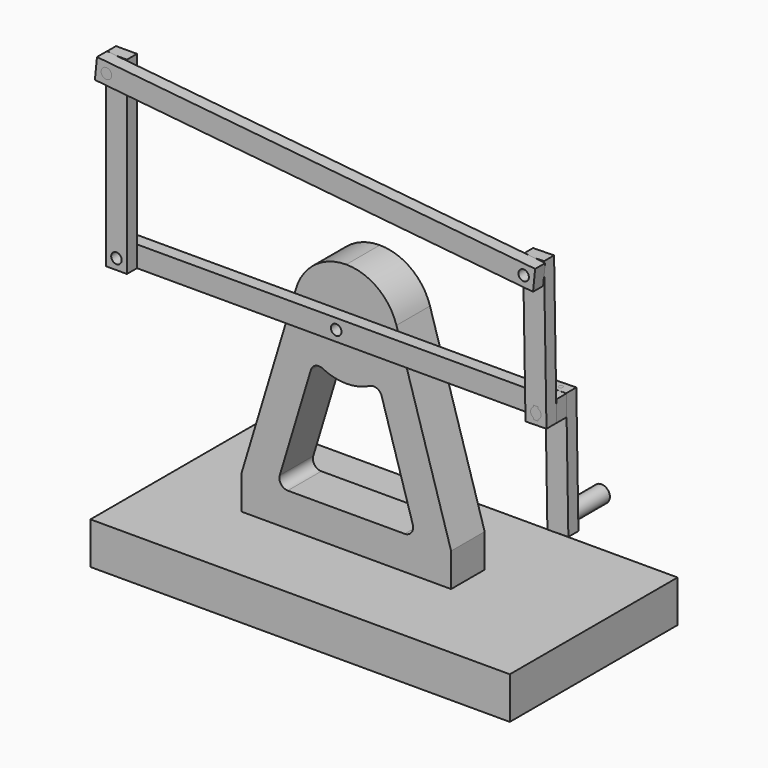
from build123d import *

# Parameters (mm, degrees)
F0_W        = 254
F0_H        = 127
F1_DEPTH    = 25.4
F3_W        = 127
F3_H        = 152.4
F4_DEPTH    = 12.7
F6_DEPTH    = 76.201
F7_R        = 5.08
F9_W        = 266.7
F9_H        = 12.7
F10_DEPTH   = 7.62
F11_W       = 12.7
F11_H       = 114.3
F12_DEPTH   = 7.62
F14_DEPTH   = 7.62
F16_DEPTH   = 7.62
F17_D       = 6.35
F17_DEPTH   = 22.861
F17_2_D     = 6.35
F17_2_DEPTH = 22.861
F17_3_D     = 6.35
F17_3_DEPTH = 22.861
F17_4_D     = 6.35
F17_4_DEPTH = 22.861
F18_D       = 6.35
F21_DEPTH   = 7.62
F22_R       = 5.08
F23_DEPTH   = 25.4
F24_R       = 3.175
F25_DEPTH   = 15.24
F26_D       = 6.35
F27_W       = 2.54
F27_H       = 7.62
F28_DEPTH   = 91.441
F30_DEPTH   = 25.4
F31_DEPTH   = 7.62
F32_W       = 2.54
F32_H       = 1.27
F33_DEPTH   = 17.78
F35_D       = 2.54
F35_DEPTH   = 7.62
F35_TIP     = 0.7630929862
F36_R       = 1.27
F37_DEPTH   = 12.7


with BuildPart() as f1:
    # F0 (on Top) → F1 (new body)
    with BuildSketch(Plane.XY):
        with Locations((127, 63.5)):
            Rectangle(F0_W, F0_H)
    extrude(amount=F1_DEPTH)


with BuildPart() as f4:
    # F3 (on mid) → F4 (new body, symmetric)
    with BuildSketch(Plane.XZ.offset(-63.5)):
        with Locations((114.3, 101.6)):
            Rectangle(F3_W, F3_H)
    extrude(amount=F4_DEPTH, both=True)

    # F5 (on face) → F6 (cut, through all)
    with BuildSketch(Plane.XZ.offset(-50.8)):
        with BuildLine():
            Line((156.5717554914, 45.72), (133.8126678121, 121.0036770193))
            ThreePointArc((133.8126678121, 121.0036770193), (114.3, 114.3), (94.7873321879, 121.0036770193))
            Line((94.7873321879, 121.0036770193), (72.0282445086, 45.72))
            Line((72.0282445086, 45.72), (156.5717554914, 45.72))
        make_face()
        with BuildLine():
            ThreePointArc((83.9084148767, 155.2377121033), (95.3744532349, 171.5428652693), (114.3, 177.8))
            Line((114.3, 177.8), (50.8, 177.8))
            Line((50.8, 177.8), (50.8, 45.72))
            Line((50.8, 45.72), (83.9084148767, 155.2377121033))
        make_face()
        with BuildLine():
            ThreePointArc((114.3, 177.8), (133.2255467651, 171.5428652693), (144.6915851233, 155.2377121033))
            Line((144.6915851233, 155.2377121033), (177.8, 45.72))
            Line((177.8, 45.72), (177.8, 177.8))
            Line((177.8, 177.8), (114.3, 177.8))
        make_face()
    extrude(amount=-F6_DEPTH, mode=Mode.SUBTRACT)

    # F7
    f7_edges = [f4.edges().sort_by_distance(p)[0] for p in [
        (72.028245, 63.5, 45.72),
        (156.571755, 63.5, 45.72),
        (94.787332, 63.5, 121.003677),
        (133.812668, 63.5, 121.003677),
    ]]
    fillet(f7_edges, radius=F7_R)

    # F18 (through all)
    with Locations(Plane.XZ.offset(-50.8)):
        with Locations((114.3, 146.05)):
            Hole(F18_D / 2)


with BuildPart() as f10:
    # F9 (on face) → F10 (new body)
    with BuildSketch(Plane.XZ.offset(-50.8)):
        with Locations((114.3, 146.05)):
            Rectangle(F9_W, F9_H)
    extrude(amount=F10_DEPTH)

    # F17 (through all, one way)
    with BuildSketch(Plane(origin=(0, 50.8, 0), x_dir=(1, 0, 0), z_dir=(0, 1, 0))):
        with Locations((-12.7, -247.65), (-12.7, -146.05), (114.3, -146.05), (241.3, -146.05), (240.025737907, -222.2393447676)):
            Circle(F17_D / 2)
    extrude(amount=-F17_DEPTH, mode=Mode.SUBTRACT)


with BuildPart() as f12:
    # F11 (on face) → F12 (new body)
    with BuildSketch(Plane.XZ.offset(-43.18)):
        with Locations((-12.7, 196.85)):
            Rectangle(F11_W, F11_H)
    extrude(amount=F12_DEPTH)

    # F17#2 (through all, one way)
    with BuildSketch(Plane(origin=(0, 50.8, 0), x_dir=(1, 0, 0), z_dir=(0, 1, 0))):
        with Locations((-12.7, -247.65), (-12.7, -146.05), (114.3, -146.05), (241.3, -146.05), (240.025737907, -222.2393447676)):
            Circle(F17_2_D / 2)
    extrude(amount=-F17_2_DEPTH, mode=Mode.SUBTRACT)


with BuildPart() as f14:
    # F13 (on face) → F14 (new body)
    with BuildSketch(Plane.XZ.offset(-35.56)):
        Polygon((-19.6534098285, 241.9671229331), (245.7086149739, 215.2859349391), (246.9791477355, 227.9222218345), (-18.3828770669, 254.6034098285), align=None)
    extrude(amount=F14_DEPTH)

    # F17#3 (through all, one way)
    with BuildSketch(Plane(origin=(0, 50.8, 0), x_dir=(1, 0, 0), z_dir=(0, 1, 0))):
        with Locations((-12.7, -247.65), (-12.7, -146.05), (114.3, -146.05), (241.3, -146.05), (240.025737907, -222.2393447676)):
            Circle(F17_3_D / 2)
    extrude(amount=-F17_3_DEPTH, mode=Mode.SUBTRACT)


with BuildPart() as f16:
    # F15 (on face) → F16 (new body)
    with BuildSketch(Plane.XZ.offset(-43.18)):
        Polygon((247.7553005717, 139.8070764438), (246.2686614633, 228.6946453393), (233.5704373353, 228.4822683238), (235.0570764438, 139.5946994283), align=None)
    extrude(amount=F16_DEPTH)

    # F17#4 (through all, one way)
    with BuildSketch(Plane(origin=(0, 50.8, 0), x_dir=(1, 0, 0), z_dir=(0, 1, 0))):
        with Locations((-12.7, -247.65), (-12.7, -146.05), (114.3, -146.05), (241.3, -146.05), (240.025737907, -222.2393447676)):
            Circle(F17_4_D / 2)
    extrude(amount=-F17_4_DEPTH, mode=Mode.SUBTRACT)

    # F27 (on face) → F28 (cut, through all)
    with BuildSketch(Plane.XZ.offset(-35.56)):
        with Locations((241.3, 146.05)):
            Rectangle(F27_W, F27_H)
    extrude(amount=-F28_DEPTH, mode=Mode.SUBTRACT)


with BuildPart() as f21:
    # F20 (on face) → F21 (new body)
    with BuildSketch(Plane(origin=(0, 50.8, 0), x_dir=(-1, 0, 0), z_dir=(0, 1, 0))):
        Polygon((-248.8171856492, 76.3159558041), (-236.1189615212, 76.1035787886), (-234.8446994283, 152.2929235562), (-247.5429235562, 152.5053005717), align=None)
    extrude(amount=F21_DEPTH)

    # F22 (on face) → F23 (join)
    with BuildSketch(Plane(origin=(0, 58.42, 0), x_dir=(-1, 0, 0), z_dir=(0, 1, 0))):
        with Locations((-242.4680735852, 83.8297672964)):
            Circle(F22_R)
    extrude(amount=F23_DEPTH)

    # F26 (through all)
    with Locations(Plane.XZ.offset(-35.56)):
        with Locations((241.3, 146.05)):
            Hole(F26_D / 2)

    # F35
    with Locations(Plane(origin=(-2.4807042479, 0, 148.3236708146), x_dir=(0.9998601676, 0, 0.0167225996), z_dir=(-0.0167225996, 0, 0.9998601676))):
        with Locations((243.7085941089, 54.61)):
            Hole(F35_D / 2, depth=F35_DEPTH)
            with Locations((0, 0, -(F35_DEPTH + F35_TIP / 2))):  # 118° drill point
                Cone(0, F35_D / 2, F35_TIP, mode=Mode.SUBTRACT)


with BuildPart() as f25:
    # F24 (on face) → F25 (new body)
    with BuildSketch(Plane.XZ.offset(-27.94)):
        with Locations((-12.7, 247.65)):
            Circle(F24_R)
    extrude(amount=-F25_DEPTH)


with BuildPart() as f30:
    # F29 (on face) → F30 (new body)
    with BuildSketch(Plane.XZ.offset(-35.56)):
        with BuildLine():
            ThreePointArc((244.475, 146.05), (243.9563955842, 147.7890191201), (242.57, 148.9599355663))
            ThreePointArc((242.57, 148.9599355663), (241.3, 149.225), (240.03, 148.9599355663))
            ThreePointArc((240.03, 148.9599355663), (238.125, 146.05), (240.03, 143.1400644337))
            ThreePointArc((240.03, 143.1400644337), (241.3, 142.875), (242.57, 143.1400644337))
            ThreePointArc((242.57, 143.1400644337), (243.9563955842, 144.3109808799), (244.475, 146.05))
        make_face()
    extrude(amount=-F30_DEPTH)

    # F29 (on face) → F31 (join)
    with BuildSketch(Plane.XZ.offset(-35.56)):
        with BuildLine():
            Line((242.57, 148.9599355663), (242.57, 149.86))
            Line((242.57, 149.86), (240.03, 149.86))
            Line((240.03, 149.86), (240.03, 148.9599355663))
            ThreePointArc((240.03, 148.9599355663), (241.3, 149.225), (242.57, 148.9599355663))
        make_face()
        with BuildLine():
            ThreePointArc((244.475, 146.05), (243.9563955842, 147.7890191201), (242.57, 148.9599355663))
            ThreePointArc((242.57, 148.9599355663), (241.3, 149.225), (240.03, 148.9599355663))
            ThreePointArc((240.03, 148.9599355663), (238.125, 146.05), (240.03, 143.1400644337))
            ThreePointArc((240.03, 143.1400644337), (241.3, 142.875), (242.57, 143.1400644337))
            ThreePointArc((242.57, 143.1400644337), (243.9563955842, 144.3109808799), (244.475, 146.05))
        make_face()
        with BuildLine():
            ThreePointArc((242.57, 143.1400644337), (241.3, 142.875), (240.03, 143.1400644337))
            Line((240.03, 143.1400644337), (240.03, 142.24))
            Line((240.03, 142.24), (242.57, 142.24))
            Line((242.57, 142.24), (242.57, 143.1400644337))
        make_face()
    extrude(amount=-F31_DEPTH)

    # F32 (on face) → F33 (cut, through all)
    with BuildSketch(Plane(origin=(0, 60.96, 0), x_dir=(-1, 0, 0), z_dir=(0, 1, 0))):
        with Locations((-241.3, 149.225)):
            Rectangle(F32_W, F32_H)
        with Locations((-241.3, 142.875)):
            Rectangle(F32_W, F32_H)
    extrude(amount=-F33_DEPTH, mode=Mode.SUBTRACT)


with BuildPart() as f37:
    # F36 (on face) → F37 (new body)
    with BuildSketch(Plane(origin=(-2.4807042479, 0, 148.3236708146), x_dir=(0.9998601676, 0, 0.0167225996), z_dir=(-0.0167225996, 0, 0.9998601676))):
        with Locations((243.7085941089, 54.61)):
            Circle(F36_R)
    extrude(amount=-F37_DEPTH)


solid = Compound([f1.part, f4.part, f10.part, f12.part, f14.part, f16.part, f21.part, f25.part, f30.part, f37.part])
